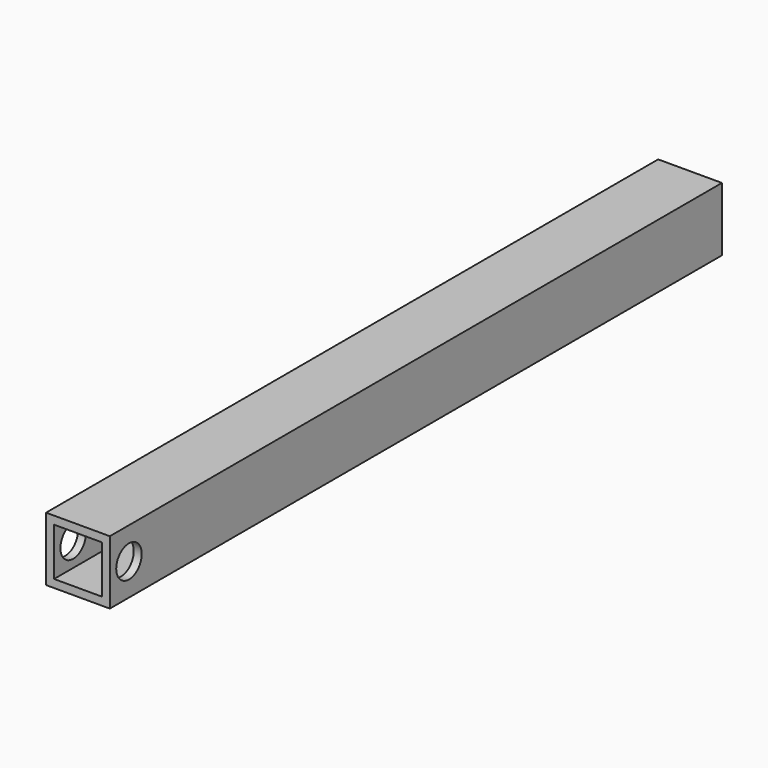
from build123d import *

# Parameters (mm, degrees)
F0_W     = 25.4
F0_H     = 25.4
F0_W_2   = 19.05
F0_H_2   = 19.05
F1_DEPTH = 304.8
F3_D     = 12.7


# Not quite as in the source:
# - a feature names something its author has since deleted; it is built from what else it names


with BuildPart() as f1:
    # F0 (on Front) → F1 (new body)
    with BuildSketch(Plane.XZ):
        with Locations((-9.525, 9.525)):
            Rectangle(F0_W, F0_H)
        with Locations((-9.525, 9.525)):
            Rectangle(F0_W_2, F0_H_2, mode=Mode.SUBTRACT)
    extrude(amount=F1_DEPTH)

    # F3 (through all)
    with Locations(Plane.YZ.offset(3.175)):
        with Locations((-295.275, 9.525)):
            Hole(F3_D / 2)


solid = f1.part
